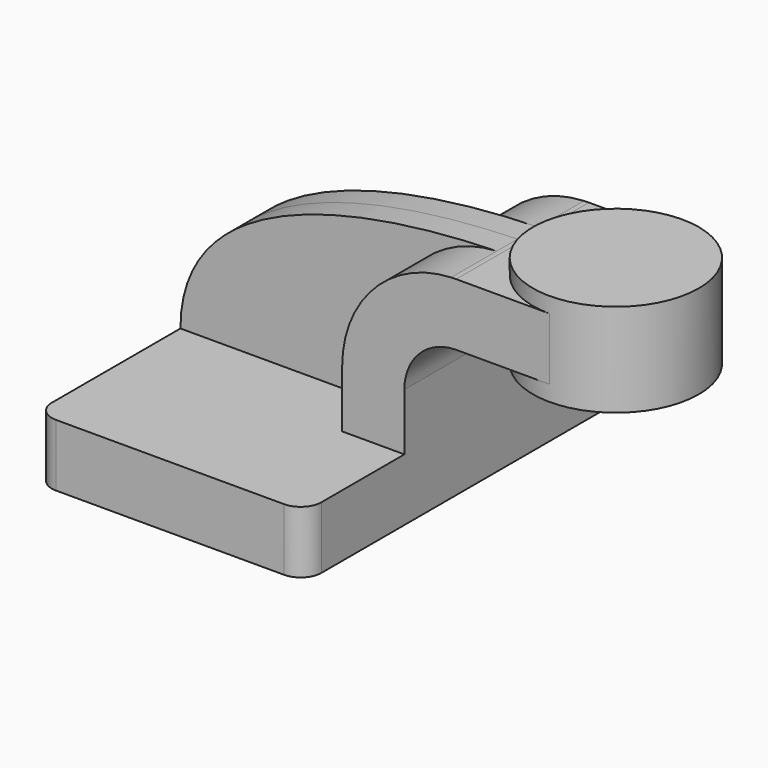
from build123d import *

# Parameters (mm, degrees)
F1_DEPTH = 63.5
F0_W     = 25.4
F0_H     = 19.05
F2_DEPTH = 25.4
F3_DEPTH = 7.9375
F5_R     = 6.35
F6_R     = 6.35


# Not quite as in the source:
# - a feature names something its author has since deleted; it is built from what else it names


with BuildPart() as f1:
    # F0 (on Front) → F1 (new body, symmetric)
    with BuildSketch(Plane.XZ):
        Polygon((22.225, 9.525), (-41.275, 9.525), (-41.275, -9.525), (41.275, -9.525), (41.275, 9.525), align=None)
    extrude(amount=F1_DEPTH, both=True)

    # F0 (on Front) → F2 (join, symmetric)
    with BuildSketch(Plane.XZ):
        with BuildLine():
            Line((22.225, 27.0002), (22.225, 9.525))
            Line((22.225, 9.525), (41.275, 9.525))
            Line((41.275, 9.525), (41.275, 27.0002))
            ThreePointArc((41.275, 27.0002), (45.9246798487, 38.2255201513), (57.15, 42.8752))
            Line((57.15, 42.8752), (60.325, 42.8752))
            Line((60.325, 42.8752), (60.325, 61.9252))
            Line((60.325, 61.9252), (57.15, 61.9252))
            add(Edge.make_bspline(
                [(55.6286861057, 61.8920504673), (56.1384142752, 61.9045266367), (56.6455676592, 61.915561496), (57.15, 61.9252)],
                knots=[110.1136190258, 110.1136190258, 110.1136190258, 110.1136190258, 111.5045361635, 111.5045361635, 111.5045361635, 111.5045361635], degree=3))
            ThreePointArc((55.6286861057, 61.8920504673), (31.9221630658, 51.1520502111), (22.225, 27.0002))
        make_face()
        with Locations((73.025, 52.4002)):
            Rectangle(F0_W, F0_H)
    extrude(amount=F2_DEPTH, both=True)

    # F0 (on Front) → F3 (join, symmetric)
    with BuildSketch(Plane.XZ):
        with BuildLine():
            add(Edge.make_bspline(
                [(-41.275, 9.525), (-41.2147135228, 50.8835652719), (15.2754458257, 60.9043595954), (55.6286861057, 61.8920504673)],
                knots=[0, 0, 0, 0, 110.1136190258, 110.1136190258, 110.1136190258, 110.1136190258], degree=3))
            Line((-41.275, 9.525), (22.225, 9.525))
            Line((22.225, 9.525), (22.225, 27.0002))
            ThreePointArc((22.225, 27.0002), (31.9221630658, 51.1520502111), (55.6286861057, 61.8920504673))
        make_face()
    extrude(amount=F3_DEPTH, both=True)

    # F0 (on Front) → F4 (revolve)
    with BuildSketch(Plane.XZ):
        Polygon((85.725, 66.675), (85.725, 61.9252), (85.725, 42.8752), (85.725, 38.1), (111.125, 38.1), (111.125, 66.675), align=None)
    revolve(axis=Axis((85.725, 0, 52.4002), (0, 0, 1)))

    # F5
    f5_edges = [f1.edges().sort_by_distance(p)[0] for p in [
        (-41.275, 63.5, 0),
    ]]
    fillet(f5_edges, radius=F5_R)

    # F6
    f6_edges = [f1.edges().sort_by_distance(p)[0] for p in [
        (-41.275, -63.5, 0),
        (41.275, 63.5, 0),
        (41.275, -63.5, 0),
    ]]
    fillet(f6_edges, radius=F6_R)


solid = f1.part
